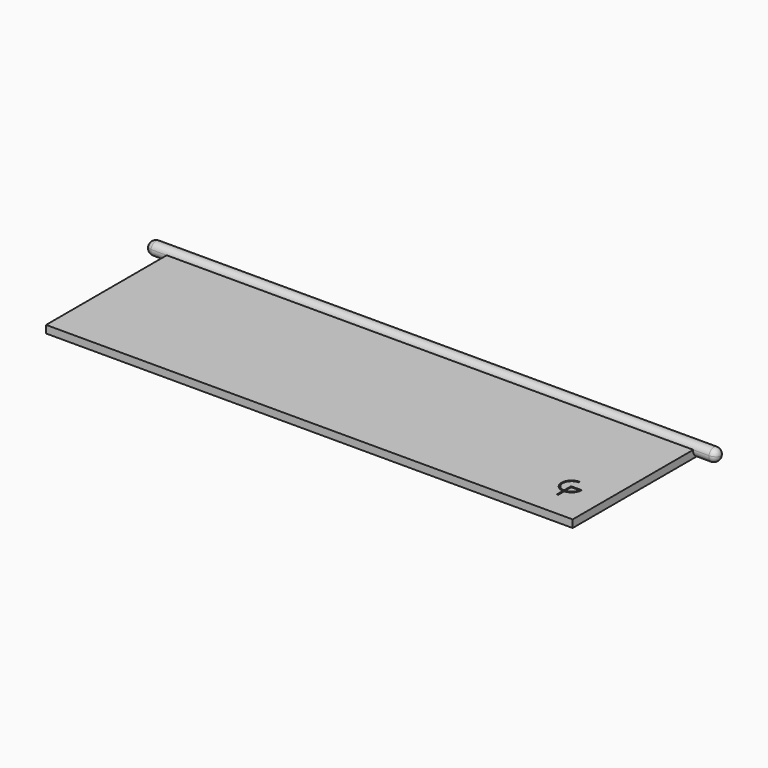
from build123d import *

# Parameters (mm, degrees)
F1_DEPTH      = 104
F2_DEPTH      = 4.3
F2_DEPTH_BACK = 108.3
F3_R          = 1.2
F5_DEPTH      = 0.5


with BuildPart() as f1:
    # F0 (on Right) → F1 (new body)
    with BuildSketch(Plane.YZ):
        with BuildLine():
            Line((-31, 0), (0, 0))
            ThreePointArc((0, 0), (-0.968246, 0.459431), (-1.224745, 1.5))
            Line((-1.224745, 1.5), (-31, 1.5))
            Line((-31, 1.5), (-31, 0))
        make_face()
    extrude(amount=-F1_DEPTH)

    # F0 (on Right) → F2 (join, two sides)
    with BuildSketch(Plane.YZ) as f2_sk:
        with BuildLine():
            ThreePointArc((-1.224745, 1.5), (-0.968246, 0.459431), (0, 0))
            Line((0, 0), (0, 1.5))
            Line((0, 1.5), (-1.224745, 1.5))
        make_face()
        with BuildLine():
            Line((0, 1.5), (0, 0))
            ThreePointArc((0, 0), (0.883883, 0.366117), (1.25, 1.25))
            ThreePointArc((1.25, 1.25), (0.125636, 2.49367), (-1.224745, 1.5))
            Line((-1.224745, 1.5), (0, 1.5))
        make_face()
    extrude(amount=F2_DEPTH)
    extrude(f2_sk.sketch, amount=-F2_DEPTH_BACK)

    # F3
    f3_edges = [f1.edges().sort_by_distance(p)[0] for p in [
        (4.3, 0, 2.5),
        (-108.3, 0, 2.5),
    ]]
    fillet(f3_edges, radius=F3_R)

    # F4 (on face) → F5 (cut)
    with BuildSketch(Plane.XY.offset(1.5)):
        with BuildLine():
            Line((-7, -20.75), (-7, -20.5))
            ThreePointArc((-7, -20.5), (-8.999099, -22.439973), (-7.12, -24.496397))
            Line((-7.12, -24.496397), (-7.12, -24.245881))
            ThreePointArc((-7.12, -24.245881), (-8.74897, -22.439965), (-7, -20.75))
        make_face()
        with BuildLine():
            Line((-7.12, -24.245881), (-7.12, -24.496397))
            ThreePointArc((-7.12, -24.496397), (-6.99499, -24.499994), (-6.87, -24.495771))
            Line((-6.87, -24.495771), (-6.87, -24.245165))
            ThreePointArc((-6.87, -24.245165), (-6.994987, -24.249993), (-7.12, -24.245881))
        make_face()
        with BuildLine():
            ThreePointArc((-6.87, -24.495771), (-6.99499, -24.499994), (-7.12, -24.496397))
            Line((-7.12, -24.496397), (-7.12, -26))
            Line((-7.12, -26), (-6.87, -26))
            Line((-6.87, -26), (-6.87, -24.495771))
        make_face()
        with BuildLine():
            Line((-6.87, -24.245165), (-6.87, -24.495771))
            ThreePointArc((-6.87, -24.495771), (-5.540548, -23.867479), (-5, -22.5))
            Line((-5, -22.5), (-5.25, -22.5))
            ThreePointArc((-5.25, -22.5), (-5.254493, -22.625322), (-5.267949, -22.75))
            ThreePointArc((-5.267949, -22.75), (-5.805978, -23.77938), (-6.87, -24.245165))
        make_face()
        with BuildLine():
            Line((-7.12, -22.5), (-7.12, -24.245881))
            ThreePointArc((-7.12, -24.245881), (-6.994987, -24.249993), (-6.87, -24.245165))
            Line((-6.87, -24.245165), (-6.87, -22.75))
            Line((-6.87, -22.75), (-5.267949, -22.75))
            ThreePointArc((-5.267949, -22.75), (-5.254493, -22.625322), (-5.25, -22.5))
            Line((-5.25, -22.5), (-7.12, -22.5))
        make_face()
    extrude(amount=-F5_DEPTH, mode=Mode.SUBTRACT)


solid = f1.part
